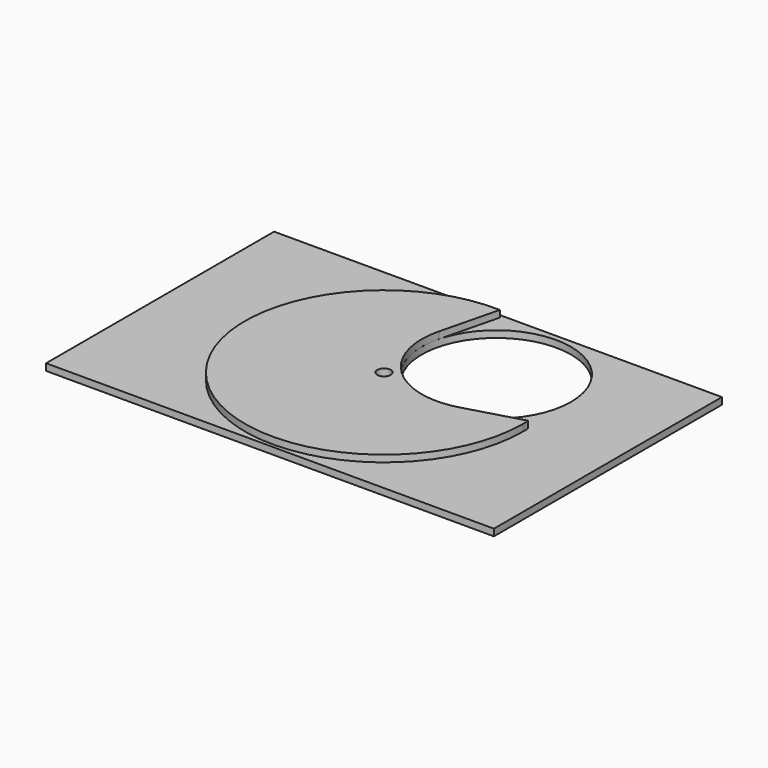
from build123d import *

# Parameters (mm, degrees)
F0_W     = 419.1
F0_H     = 266.7
F0_R     = 6.35
F1_DEPTH = 6.35
F2_R     = 69.85
F3_DEPTH = 6.35
F4_R     = 6.35
F5_DEPTH = 6.35
F6_DEPTH = 25.4
F8_DEPTH = 25.4


with BuildPart() as f1:
    # F0 (on Top) → F1 (new body)
    with BuildSketch(Plane.XY):
        Rectangle(F0_W, F0_H)
        Circle(F0_R, mode=Mode.SUBTRACT)
    extrude(amount=F1_DEPTH)

    # F2 (on face) → F3 (cut, through all)
    with BuildSketch(Plane.XY.offset(6.35)):
        with Locations((58.42, 58.42)):
            Circle(F2_R)
    extrude(amount=-F3_DEPTH, mode=Mode.SUBTRACT)


with BuildPart() as f5:
    # F4 (on face) → F5 (new body)
    with BuildSketch(Plane.XY.offset(6.35)):
        with BuildLine():
            ThreePointArc((36.8406854071, 124.8530917668), (-104.2623298413, -77.9416268823), (130.175, 0))
            ThreePointArc((130.175, 0), (128.8376533583, 18.6115475479), (124.8530917668, 36.8406854071))
            ThreePointArc((124.8530917668, 36.8406854071), (9.0285913341, 9.0285913341), (36.8406854071, 124.8530917668))
        make_face()
        Circle(F4_R, mode=Mode.SUBTRACT)
        with BuildLine():
            ThreePointArc((36.8406854071, 124.8530917668), (9.0285913341, 9.0285913341), (124.8530917668, 36.8406854071))
            ThreePointArc((124.8530917668, 36.8406854071), (92.047625241, 92.047625241), (36.8406854071, 124.8530917668))
        make_face()
    extrude(amount=F5_DEPTH)

    # F2 (on face) → F6 (cut)
    with BuildSketch(Plane.XY.offset(6.35)):
        with Locations((58.42, 58.42)):
            Circle(F2_R)
    extrude(amount=F6_DEPTH, mode=Mode.SUBTRACT)

    # F7 (on face) → F8 (cut)
    with BuildSketch(Plane.XY.offset(12.7)):
        with BuildLine():
            ThreePointArc((36.8406854071, 124.8530917668), (7.481865656, 106.2146541943), (-9.2512492182, 75.7296657751))
            Line((-9.2512492182, 75.7296657751), (36.8406854071, 65.8533647656))
            Line((36.8406854071, 65.8533647656), (49.260482192, 140.2665227652))
            Line((49.260482192, 140.2665227652), (4.2698969352, 130.1049522699))
            ThreePointArc((4.2698969352, 130.1049522699), (20.7223431305, 128.5150384982), (36.8406854071, 124.8530917668))
        make_face()
        with BuildLine():
            Line((4.2698969352, 130.1049522699), (-9.2512492182, 75.7296657751))
            ThreePointArc((-9.2512492182, 75.7296657751), (7.481865656, 106.2146541943), (36.8406854071, 124.8530917668))
            ThreePointArc((36.8406854071, 124.8530917668), (20.7223431305, 128.5150384982), (4.2698969352, 130.1049522699))
        make_face()
        with BuildLine():
            Line((127.2549563477, 54.1487200117), (75.5184735859, -9.3049193505))
            Line((75.5184735859, -9.3049193505), (79.4723410938, -8.1819626923))
            ThreePointArc((79.4723410938, -8.1819626923), (107.6153753027, 8.833332953), (124.8530917668, 36.8406854071))
            ThreePointArc((124.8530917668, 36.8406854071), (128.3596935609, 21.6637876178), (130.0283778221, 6.1766970102))
            Line((130.0283778221, 6.1766970103), (140.0697380304, 9.0285913341))
            Line((140.0697380304, 9.0285913341), (127.2549563477, 54.1487200117))
        make_face()
        with BuildLine():
            Line((79.4723410938, -8.1819626923), (130.0283778221, 6.1766970103))
            ThreePointArc((130.0283778221, 6.1766970102), (128.3596935609, 21.6637876178), (124.8530917668, 36.8406854071))
            ThreePointArc((124.8530917668, 36.8406854071), (107.6153753027, 8.833332953), (79.4723410938, -8.1819626923))
        make_face()
    extrude(amount=-F8_DEPTH, mode=Mode.SUBTRACT)


solid = Compound([f1.part, f5.part])
